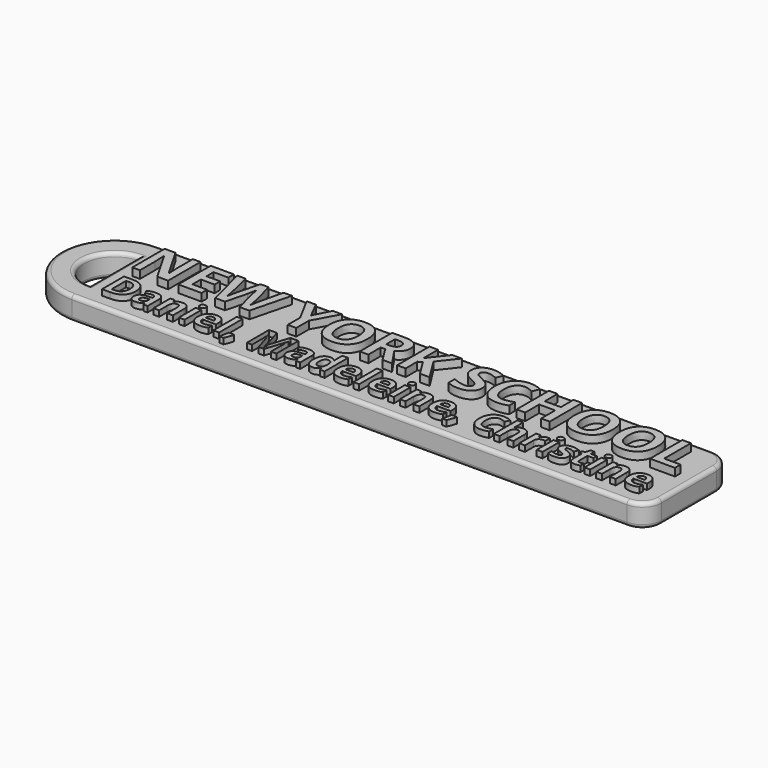
from build123d import *

# Parameters (mm, degrees)
F0_W         = 75
F0_H         = 14
F1_DEPTH     = 3
F2_TEXT_SIZE = 7.388878199
F3_DEPTH     = 1
F4_TEXT_SIZE = 5.0420541044
F5_DEPTH     = 0.75
F7_DEPTH     = 3
F8_R         = 2.5
F9_R         = 0.5


# Not quite as in the source:
# - Text() gives the source's letters only with a copy of the font that has no kerning and outlines rounded to 1/6400 em; it was checked with that copy


with BuildPart() as f1:
    # F0 (on Top) → F1 (new body)
    with BuildSketch(Plane.XY):
        Rectangle(F0_W, F0_H)
    extrude(amount=F1_DEPTH)

    # F2 (on face) → F3 (join)
    with BuildSketch(Plane.XY.offset(3)):
        with Locations((-36, 0.1800076967)):
            Text('NEW YORK SCHOOL', F2_TEXT_SIZE, font='Open Sans', font_style=FontStyle.BOLD, text_align=(TextAlign.LEFT, TextAlign.BOTTOM))
    extrude(amount=F3_DEPTH)

    # F4 (on face) → F5 (join)
    with BuildSketch(Plane.XY.offset(3)):
        with Locations((-35.5, -5.1302789552)):
            Text('Daniel, Madeleine, Christine', F4_TEXT_SIZE, font='Open Sans', font_style=FontStyle.BOLD, text_align=(TextAlign.LEFT, TextAlign.BOTTOM))
    extrude(amount=F5_DEPTH)

    # F6 (on face) → F7 (join)
    with BuildSketch(Plane.XY.offset(3)):
        with BuildLine():
            Line((-37.5, 4), (-37.5, 7))
            ThreePointArc((-37.5, 7), (-44.5, 0), (-37.5, -7))
            Line((-37.5, -7), (-37.5, -4))
            ThreePointArc((-37.5, -4), (-41.5, 0), (-37.5, 4))
        make_face()
    extrude(amount=-F7_DEPTH)

    # F8
    f8_edges = [f1.edges().sort_by_distance(p)[0] for p in [
        (37.5, 7, 1.5),
        (37.5, -7, 1.5),
    ]]
    fillet(f8_edges, radius=F8_R)

    # F9
    f9_edges = [f1.edges().sort_by_distance(p)[0] for p in [
        (-41.5, 0, 3),
        (-37.5, 0, 3),
        (-1.25, 7, 3),
        (-41.5, 0, 0),
        (-44.5, 0, 0),
        (-37.5, 0, 0),
    ]]
    fillet(f9_edges, radius=F9_R)


solid = f1.part
